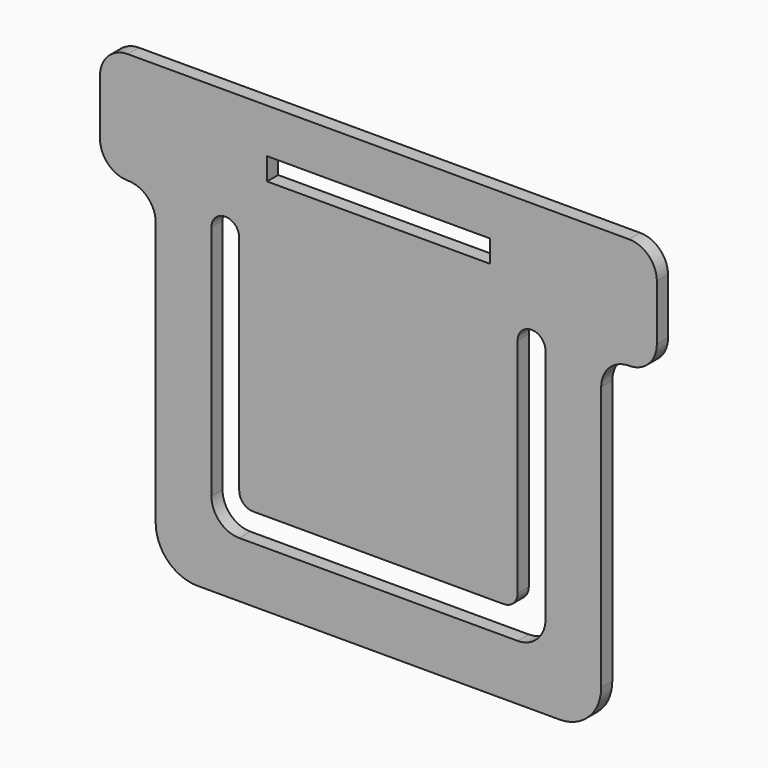
from build123d import *

# Parameters (mm, degrees)
F0_W      = 25.4
F0_H      = 19.05
F1_DEPTH  = 0.79375
F2_R      = 2.38125
F3_W      = 19.05
F3_H      = 15.875
F4_DEPTH  = 4.9276
F5_W      = 12.7
F5_H      = 1.27
F6_DEPTH  = 0.79375
F7_R      = 1.58749
F8_R      = 1.5875
F9_W      = 12.7
F9_H      = 1.27
F9_W_2    = 15.875
F9_H_2    = 14.2875
F10_DEPTH = 0.79375
F11_R     = 0.79374
F12_R     = 0.79375


# Not quite as in the source:
# - a fillet or chamfer is up to 0.001 mm smaller than in the source, because OpenCascade refuses the exact size
# - ends of sketch curves that miss each other by under 0.0002 mm in the source are joined


with BuildPart() as f1:
    # F0 (on Front) → F1 (new body)
    with BuildSketch(Plane.XZ):
        Rectangle(F0_W, F0_H)
    extrude(amount=F1_DEPTH)

    # F2
    f2_edges = [f1.edges().sort_by_distance(p)[0] for p in [
        (12.7, -0.396875, -9.525),
        (-12.7, -0.396875, -9.525),
    ]]
    fillet(f2_edges, radius=F2_R)

    # F3 (on face) → F4 (cut)
    with BuildSketch(Plane.XZ.offset(0.79375)):
        with Locations((0, 1.5875)):
            Rectangle(F3_W, F3_H)
    extrude(amount=-F4_DEPTH, mode=Mode.SUBTRACT)

    # F5 (on face) → F6 (join)
    with BuildSketch(Plane.XZ.offset(0.79375)):
        Polygon((-15.875, 15.875), (-15.875, 9.525), (-12.7, 9.525), (-9.525, 9.525), (9.525, 9.525), (12.7, 9.525), (15.875, 9.525), (15.875, 15.875), align=None)
        with Locations((0, 12.7)):
            Rectangle(F5_W, F5_H, mode=Mode.SUBTRACT)
    extrude(amount=-F6_DEPTH)

    # F7 (radius 1.5875 in the source; OpenCascade refuses exactly that, so slightly less here)
    f7_edges = [f1.edges().sort_by_distance(p)[0] for p in [
        (-15.875, -0.396875, 15.875),
        (15.875, -0.396875, 15.875),
        (15.875, -0.396875, 9.525),
        (12.7, -0.396875, 9.525),
        (-15.875, -0.396875, 9.525),
        (-12.7, -0.396875, 9.525),
    ]]
    fillet(f7_edges, radius=F7_R)

    # F8
    f8_edges = [f1.edges().sort_by_distance(p)[0] for p in [
        (-9.525, -0.396875, -6.35),
        (9.525, -0.396875, -6.35),
    ]]
    fillet(f8_edges, radius=F8_R)

    # F9 (on face) → F10 (join)
    with BuildSketch(Plane.XZ.offset(0.79375)):
        with BuildLine():
            ThreePointArc((-14.28751, 15.875), (-15.4100349441, 15.4100349441), (-15.875, 14.28751))
            Line((-15.875, 14.28751), (-15.875, 11.11249))
            ThreePointArc((-15.875, 11.11249), (-15.4100349441, 9.9899650559), (-14.28751, 9.525))
            ThreePointArc((-14.28751, 9.525), (-13.1649650559, 9.0600349441), (-12.7, 7.93751))
            Line((-12.7, 7.93751), (-12.7, -7.14375))
            ThreePointArc((-12.7, -7.14375), (-12.0025480227, -8.8275480227), (-10.31875, -9.525))
            Line((-10.31875, -9.525), (10.31875, -9.525))
            ThreePointArc((10.31875, -9.525), (12.0025480227, -8.8275480227), (12.7, -7.14375))
            Line((12.7, -7.14375), (12.7, 7.93751))
            ThreePointArc((12.7, 7.93751), (13.1649650559, 9.0600349441), (14.28749, 9.525))
            ThreePointArc((14.28749, 9.525), (15.4100349441, 9.9899650559), (15.875, 11.11249))
            Line((15.875, 11.11249), (15.875, 14.28751))
            ThreePointArc((15.875, 14.28751), (15.4100349441, 15.4100349441), (14.28751, 15.875))
            Line((14.28751, 15.875), (-14.28751, 15.875))
        make_face()
        with BuildLine():
            Line((-9.525, 9.525), (-7.9375, 9.525))
            Line((-7.9375, 9.525), (7.9375, 9.525))
            Line((7.9375, 9.525), (9.525, 9.525))
            Line((9.525, 9.525), (9.525, -4.7625))
            ThreePointArc((9.525, -4.7625), (9.0600320151, -5.8850320151), (7.9375, -6.35))
            Line((7.9375, -6.35), (-7.9375, -6.35))
            ThreePointArc((-7.9375, -6.35), (-9.0600320151, -5.8850320151), (-9.525, -4.7625))
            Line((-9.525, -4.7625), (-9.525, 9.525))
        make_face(mode=Mode.SUBTRACT)
        with Locations((0, 12.7)):
            Rectangle(F9_W, F9_H, mode=Mode.SUBTRACT)
        with Locations((0, 2.38125)):
            Rectangle(F9_W_2, F9_H_2)
    extrude(amount=-F10_DEPTH)

    # F11 (radius 0.79375 in the source; OpenCascade refuses exactly that, so slightly less here)
    f11_edges = [f1.edges().sort_by_distance(p)[0] for p in [
        (-7.9375, -0.396875, 9.525),
        (-9.525, -0.396875, 9.525),
        (7.9375, -0.396875, 9.525),
        (9.525, -0.396875, 9.525),
    ]]
    fillet(f11_edges, radius=F11_R)

    # F12
    f12_edges = [f1.edges().sort_by_distance(p)[0] for p in [
        (-7.9375, -0.396875, -4.7625),
        (7.9375, -0.396875, -4.7625),
    ]]
    fillet(f12_edges, radius=F12_R)


solid = f1.part
